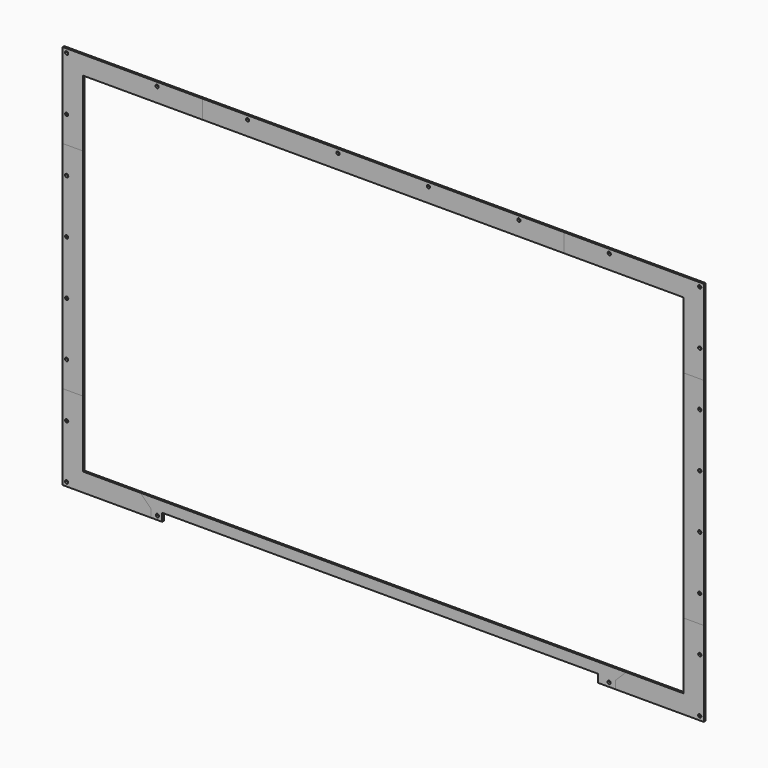
from build123d import *

# Parameters (mm, degrees)
F0_R     = 2.54
F1_DEPTH = 1.5875
F0_W     = 573.314286
F0_H     = 16.66875
F2_DEPTH = 1.5875
F3_DEPTH = 1.5875
F0_W_2   = 19.304
F0_H_2   = 341.992858
F0_W_3   = 12.7
F4_DEPTH = 1.5875
F5_DEPTH = 1.5875
F0_W_4   = 28.00096
F0_H_3   = 12.7
F0_W_5   = 18.00098
F6_DEPTH = 1.5875
F7_DEPTH = 1.5875
F8_DEPTH = 1.5875


# Not quite as in the source:
# - a feature names something its author has since deleted; it is built from what else it names


with BuildPart() as f1:
    # F0 (on Front) → F1 (new body, symmetric)
    with BuildSketch(Plane.XZ):
        Polygon((-286.657143, 276.225), (-286.657143, 292.89375), (-495.3, 292.89375), (-495.3, 170.996429), (-475.996, 170.996429), (-475.996, 276.225), align=None)
        with BuildLine():
            Line((-495.3, 170.996429), (-495.3, 292.89375))
            Line((-495.3, 292.89375), (-499.853949, 297.447699))
            ThreePointArc((-499.853949, 297.447699), (-503.446051, 297.447699), (-503.446051, 301.039801))
            Line((-503.446051, 301.039801), (-508, 305.59375))
            Line((-508, 305.59375), (-508, 170.996429))
            Line((-508, 170.996429), (-501.65, 170.996429))
            Line((-501.65, 170.996429), (-495.3, 170.996429))
        make_face()
        with BuildLine():
            ThreePointArc((-499.11, 213.745536), (-499.853949, 211.949484), (-501.65, 211.205536))
            ThreePointArc((-501.65, 211.205536), (-503.446051, 215.541587), (-499.11, 213.745536))
        make_face(mode=Mode.SUBTRACT)
        with BuildLine():
            Line((-495.3, 292.89375), (-286.657143, 292.89375))
            Line((-286.657143, 292.89375), (-286.657143, 299.24375))
            Line((-286.657143, 299.24375), (-286.657143, 305.59375))
            Line((-286.657143, 305.59375), (-508, 305.59375))
            Line((-508, 305.59375), (-503.446051, 301.039801))
            ThreePointArc((-503.446051, 301.039801), (-500.677984, 301.590404), (-499.11, 299.24375))
            ThreePointArc((-499.11, 299.24375), (-499.303346, 298.271734), (-499.853949, 297.447699))
            Line((-499.853949, 297.447699), (-495.3, 292.89375))
        make_face()
        with Locations((-358.321429, 299.24375)):
            Circle(F0_R, mode=Mode.SUBTRACT)
    extrude(amount=F1_DEPTH, both=True)


with BuildPart() as f2:
    # F0 (on Front) → F2 (new body, symmetric)
    with BuildSketch(Plane.XZ):
        with Locations((0, 284.559375)):
            Rectangle(F0_W, F0_H)
        Polygon((-286.657143, 292.89375), (286.657143, 292.89375), (286.657143, 305.59375), (-286.657143, 305.59375), (-286.657143, 299.24375), align=None)
        with BuildLine():
            ThreePointArc((-212.452857, 299.24375), (-214.992857, 296.70375), (-217.532857, 299.24375))
            ThreePointArc((-217.532857, 299.24375), (-214.992857, 301.78375), (-212.452857, 299.24375))
        make_face(mode=Mode.SUBTRACT)
        with Locations((-71.664286, 299.24375)):
            Circle(F0_R, mode=Mode.SUBTRACT)
        with Locations((71.664286, 299.24375)):
            Circle(F0_R, mode=Mode.SUBTRACT)
        with Locations((214.992857, 299.24375)):
            Circle(F0_R, mode=Mode.SUBTRACT)
    extrude(amount=F2_DEPTH, both=True)


with BuildPart() as f3:
    # F0 (on Front) → F3 (new body, symmetric)
    with BuildSketch(Plane.XZ):
        Polygon((495.3, 170.996429), (495.3, 292.89375), (286.657143, 292.89375), (286.657143, 276.225), (475.996, 276.225), (475.996, 170.996429), align=None)
        Polygon((286.657143, 292.89375), (495.3, 292.89375), (495.3, 170.996429), (508, 170.996429), (508, 305.59375), (286.657143, 305.59375), align=None)
        with Locations((501.65, 213.745536)):
            Circle(F0_R, mode=Mode.SUBTRACT)
        with Locations((358.321429, 299.24375)):
            Circle(F0_R, mode=Mode.SUBTRACT)
        with Locations((501.65, 299.24375)):
            Circle(F0_R, mode=Mode.SUBTRACT)
    extrude(amount=F3_DEPTH, both=True)


with BuildPart() as f4:
    # F0 (on Front) → F4 (new body, symmetric)
    with BuildSketch(Plane.XZ):
        with Locations((485.648, 0)):
            Rectangle(F0_W_2, F0_H_2)
        with Locations((501.65, 0)):
            Rectangle(F0_W_3, F0_H_2)
        with Locations((501.65, -128.247321)):
            Circle(F0_R, mode=Mode.SUBTRACT)
        with Locations((501.65, -42.749107)):
            Circle(F0_R, mode=Mode.SUBTRACT)
        with Locations((501.65, 42.749107)):
            Circle(F0_R, mode=Mode.SUBTRACT)
        with Locations((501.65, 128.247321)):
            Circle(F0_R, mode=Mode.SUBTRACT)
    extrude(amount=F4_DEPTH, both=True)


with BuildPart() as f5:
    # F0 (on Front) → F5 (new body, symmetric)
    with BuildSketch(Plane.XZ):
        Polygon((508, -170.996429), (495.3, -170.996429), (495.3, -292.89375), (368.3, -292.89375), (368.3, -305.59375), (508, -305.59375), align=None)
        with Locations((501.65, -299.24375)):
            Circle(F0_R, mode=Mode.SUBTRACT)
        with Locations((501.65, -213.745536)):
            Circle(F0_R, mode=Mode.SUBTRACT)
        Polygon((495.3, -292.89375), (495.3, -170.996429), (475.996, -170.996429), (475.996, -276.225), (384.96875, -276.225), (368.3, -292.89375), align=None)
    extrude(amount=F5_DEPTH, both=True)


with BuildPart() as f6:
    # F0 (on Front) → F6 (new body, symmetric)
    with BuildSketch(Plane.XZ):
        Polygon((340.29904, -292.89375), (368.3, -292.89375), (384.96875, -276.225), (-384.96875, -276.225), (-368.3, -292.89375), (-350.29902, -292.89375), align=None)
        with Locations((354.29952, -299.24375)):
            Rectangle(F0_W_4, F0_H_3)
        with Locations((357.84, -299.24375)):
            Circle(F0_R, mode=Mode.SUBTRACT)
        with Locations((-359.29951, -299.24375)):
            Rectangle(F0_W_5, F0_H_3)
        with Locations((-357.84, -299.24375)):
            Circle(F0_R, mode=Mode.SUBTRACT)
    extrude(amount=F6_DEPTH, both=True)


with BuildPart() as f7:
    # F0 (on Front) → F7 (new body, symmetric)
    with BuildSketch(Plane.XZ):
        with BuildLine():
            Line((-368.3, -292.89375), (-495.3, -292.89375))
            Line((-495.3, -292.89375), (-499.853949, -297.447699))
            ThreePointArc((-499.853949, -297.447699), (-499.303346, -298.271734), (-499.11, -299.24375))
            ThreePointArc((-499.11, -299.24375), (-500.677984, -301.590404), (-503.446051, -301.039801))
            Line((-503.446051, -301.039801), (-508, -305.59375))
            Line((-508, -305.59375), (-368.3, -305.59375))
            Line((-368.3, -305.59375), (-368.3, -292.89375))
        make_face()
        with BuildLine():
            Line((-495.3, -292.89375), (-495.3, -170.996429))
            Line((-495.3, -170.996429), (-508, -170.996429))
            Line((-508, -170.996429), (-508, -305.59375))
            Line((-508, -305.59375), (-503.446051, -301.039801))
            ThreePointArc((-503.446051, -301.039801), (-503.446051, -297.447699), (-499.853949, -297.447699))
            Line((-499.853949, -297.447699), (-495.3, -292.89375))
        make_face()
        with Locations((-501.65, -213.745536)):
            Circle(F0_R, mode=Mode.SUBTRACT)
        Polygon((-475.996, -170.996429), (-495.3, -170.996429), (-495.3, -292.89375), (-368.3, -292.89375), (-384.96875, -276.225), (-475.996, -276.225), align=None)
    extrude(amount=F7_DEPTH, both=True)


with BuildPart() as f8:
    # F0 (on Front) → F8 (new body, symmetric)
    with BuildSketch(Plane.XZ):
        with Locations((-485.648, 0)):
            Rectangle(F0_W_2, F0_H_2)
        Polygon((-495.3, -170.996429), (-495.3, 170.996429), (-501.65, 170.996429), (-508, 170.996429), (-508, -170.996429), align=None)
        with Locations((-501.65, -128.247321)):
            Circle(F0_R, mode=Mode.SUBTRACT)
        with Locations((-501.65, -42.749107)):
            Circle(F0_R, mode=Mode.SUBTRACT)
        with Locations((-501.65, 42.749107)):
            Circle(F0_R, mode=Mode.SUBTRACT)
        with BuildLine():
            ThreePointArc((-499.11, 128.247321), (-503.446051, 126.45127), (-501.65, 130.787321))
            ThreePointArc((-501.65, 130.787321), (-499.853949, 130.043373), (-499.11, 128.247321))
        make_face(mode=Mode.SUBTRACT)
    extrude(amount=F8_DEPTH, both=True)


solid = Compound([f1.part, f2.part, f3.part, f4.part, f5.part, f6.part, f7.part, f8.part])
